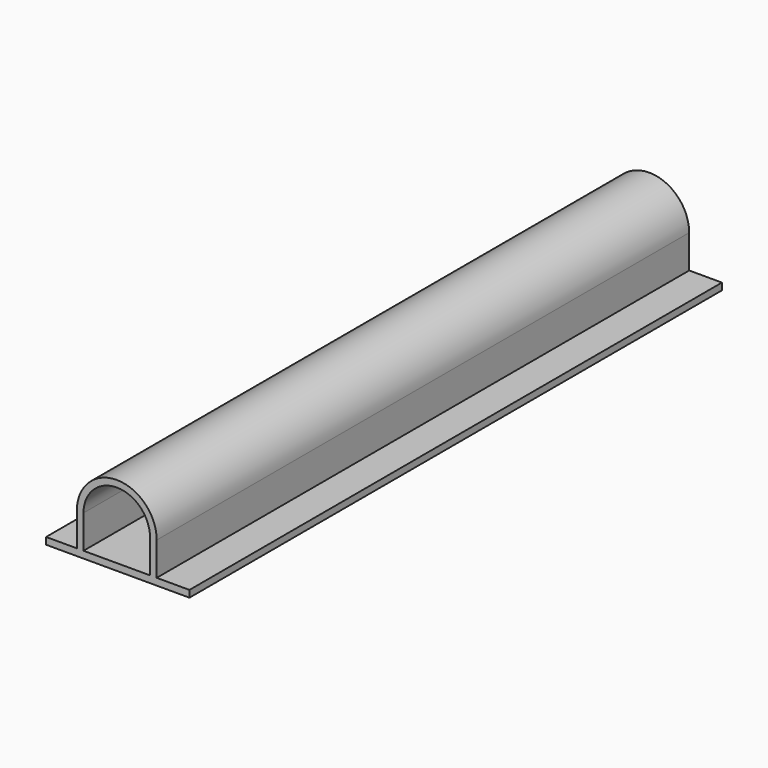
from build123d import *

# Parameters (mm, degrees)
F0_W     = 0.25
F0_H     = 1.25
F1_DEPTH = 25


# Not quite as in the source:
# - a feature names something its author has since deleted; it is built from what else it names


with BuildPart() as f1:
    # F0 (on Front) → F1 (new body)
    with BuildSketch(Plane.XZ):
        with BuildLine():
            ThreePointArc((-1.25, 0), (0, 1.25), (1.25, 0))
            Line((1.25, 0), (1.5, 0))
            ThreePointArc((1.5, 0), (0, 1.5), (-1.5, 0))
            Line((-1.5, 0), (-1.25, 0))
        make_face()
        with Locations((1.375, -0.625)):
            Rectangle(F0_W, F0_H)
        with Locations((-1.375, -0.625)):
            Rectangle(F0_W, F0_H)
        Polygon((1.5, -1.25), (1.25, -1.25), (-1.25, -1.25), (-1.5, -1.25), (-2.6555589866, -1.25), (-2.6555589866, -1.5083510661), (2.7294615284, -1.5083510661), (2.7294615284, -1.25), align=None)
    extrude(amount=F1_DEPTH)


solid = f1.part
